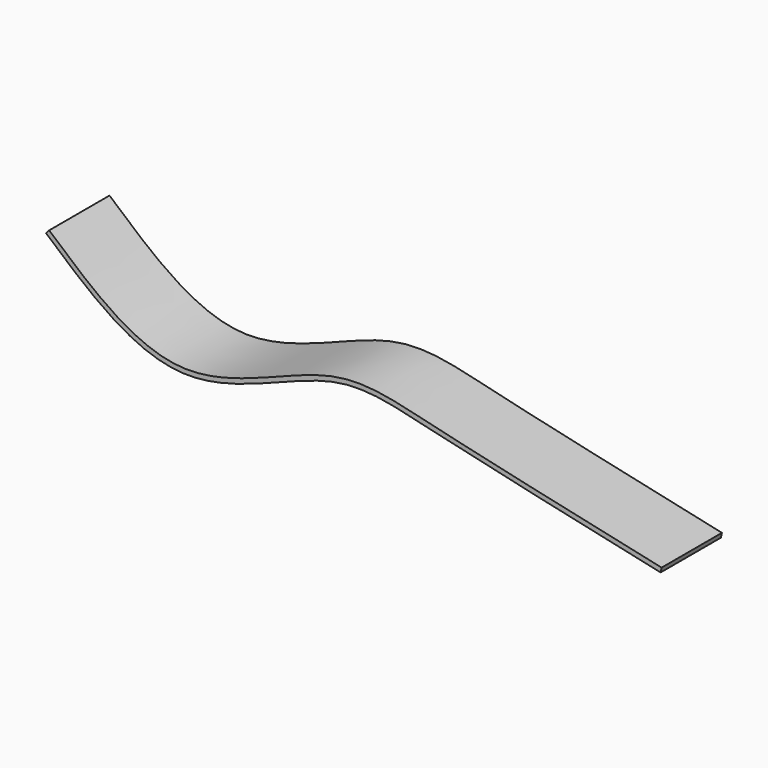
from build123d import *

# Parameters (mm, degrees)
F1_DEPTH = 20.32


# Not quite as in the source:
# - the dataset's text gives a spline's control points without its knots; the knots are read off the source's solid


with BuildPart() as f1:
    # F0 (on Front) → F1 (new body)
    with BuildSketch(Plane.XZ):
        with BuildLine():
            add(Edge.make_bspline(
                [(0, 0), (11.6153431161, -10.1995846502), (34.5990776533, -30.3819024387), (75.6615524149, -5.5061938715), (103.1369708354, -12.952782874), (141.7235298137, -21.2981937577), (165.1, -26.35400215)],
                knots=[0, 0, 0, 0, 0.2486917687, 0.4920961469, 0.6923022007, 1, 1, 1, 1], degree=3))
            Line((0, 0), (-0.8379821345, -0.9542986652))
            add(Edge.make_bspline(
                [(-0.8379821345, -0.9542986652), (2.0811291358, -3.5176084363), (7.9402091462, -8.6630340429), (15.45350657, -14.3757113466), (21.6769271533, -18.0476862634), (26.4779227998, -20.2306343273), (30.6110762277, -21.4673248765), (34.0026618164, -22.0404748308), (36.592973535, -22.2449703031), (39.2127446959, -22.2100254196), (42.7216460296, -21.884251651), (47.1267953576, -21.0221521093), (52.3944970254, -19.4722009884), (57.5963521975, -17.60940142), (62.6795215662, -15.6324267191), (66.7682177009, -14.0539926691), (69.918386264, -12.9303950215), (72.2112643931, -12.1816878562), (74.4259966202, -11.5497969896), (76.5475427612, -11.0615791003), (78.597647512, -10.7178430671), (81.2596795514, -10.4337459872), (84.4963410052, -10.3806224531), (88.3729017419, -10.7223823464), (92.3704661766, -11.3975449924), (96.6075013598, -12.3304399956), (101.1959541423, -13.4431571249), (106.2489596032, -14.643984179), (113.5366783666, -16.33212648), (123.5670527853, -18.5957219616), (136.7083354505, -21.4940887172), (150.5862403185, -24.5143706598), (160.0832737225, -26.5683596311), (164.831534484, -27.5953023823)],
                knots=[0, 0, 0, 0, 0.0625, 0.125, 0.15625, 0.1875, 0.21875, 0.234375, 0.25, 0.265625, 0.28125, 0.3125, 0.34375, 0.375, 0.40625, 0.4375, 0.453125, 0.46875, 0.484375, 0.5, 0.515625, 0.53125, 0.5625, 0.59375, 0.625, 0.65625, 0.6875, 0.71875, 0.75, 0.8125, 0.875, 0.9375, 1, 1, 1, 1], degree=3))
            Line((164.831534484, -27.5953023823), (165.1, -26.35400215))
        make_face()
    extrude(amount=F1_DEPTH)


solid = f1.part
